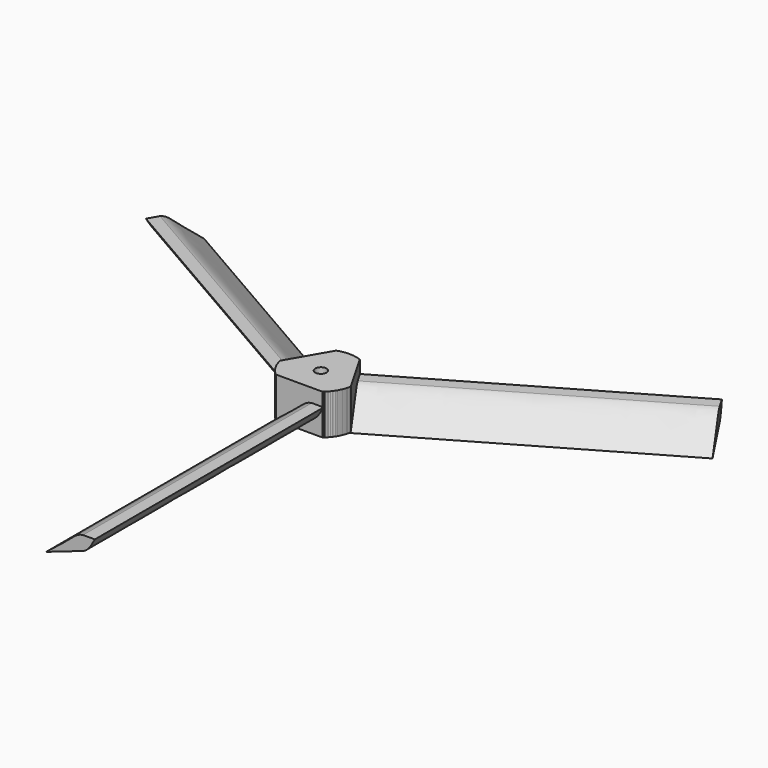
from build123d import *

# Parameters (mm, degrees)
F0_R     = 6.35
F0_R_2   = 0.99949
F1_DEPTH = 9.525
F4_DEPTH = 25.4
F6_DEPTH = 50.8
F7_COUNT = 3
F8_W     = 8.2890069642
F8_H     = 2.380754333
F9_DEPTH = 25.4


with BuildPart() as f1:
    # F0 (on Top) → F1 (new body)
    with BuildSketch(Plane.XY):
        Circle(F0_R)
        Circle(F0_R_2, mode=Mode.SUBTRACT)
    extrude(amount=F1_DEPTH)

    # F3 (on offset) → F4 (cut)
    with BuildSketch(Plane.XY.offset(9.525)):
        Polygon((-19.2380820383, -11.0045537162), (19.2410791448, -11.0045537162), (0.0014985533, 22.3193773847), align=None)
        Polygon((0.0014985533, 9.6193773847), (8.2425565167, -4.6545537162), (-8.2395594102, -4.6545537162), (-8.2425565167, -4.6545537162), (0, 9.621972955), align=None, mode=Mode.SUBTRACT)
    extrude(amount=-F4_DEPTH, mode=Mode.SUBTRACT)

    # F5 (on face) → F6 (join)
    with BuildSketch(Plane.XZ.offset(4.6545537162)):
        with BuildLine():
            add(Edge.make_bspline(
                [(4.319447847, 7.14375), (3.8768217141, 6.3398531681), (3.0702504394, 4.8749597867), (1.3331871276, 4.307573582), (-1.2552066512, 3.4811706955), (-3.2623562204, 2.7606969439), (-4.319447847, 2.38125)],
                knots=[0, 0, 0, 0, 0.2497283334, 0.4550650881, 0.7130028867, 1, 1, 1, 1], degree=3))
            Line((4.319447847, 7.14375), (2.2289671052, 7.14375))
            add(Edge.make_bspline(
                [(2.2289671052, 7.14375), (2.0794537401, 7.1223183312), (1.3375273881, 6.9699970017), (0.3270313355, 6.1326811809), (-1.7535535369, 4.3851427196), (-3.4342742537, 3.0725461739), (-4.319447847, 2.38125)],
                knots=[0.2009623726, 0.2009623726, 0.2009623726, 0.2009623726, 0.2497283334, 0.4550650881, 0.7130028867, 1, 1, 1, 1], degree=3))
        make_face()
    extrude(amount=F6_DEPTH)


with BuildPart() as f7_1:
    # F7: instance of F1
    add(f1.part.rotate(Axis((0, 0, 9.525), (0, 0, 1)), 1 * 360 / F7_COUNT))


with BuildPart() as f7_2:
    # F7: instance of F1
    add(f1.part.rotate(Axis((0, 0, 9.525), (0, 0, 1)), 2 * 360 / F7_COUNT))


with BuildPart() as f9_tool:
    # F8 (on face) → F9 (new body)
    with BuildSketch(Plane.XZ.offset(4.8109864775)):
        Polygon((-4.1445034821, 2.380754333), (-6.2417029403, 2.380754333), (-6.2417029403, -0.2239797032), (6.5267146565, -0.2239797032), (6.5267146565, 2.380754333), (4.1445034821, 2.380754333), (4.1445034821, 0), (-4.1445034821, 0), align=None)
        with Locations((0, 1.1903771665)):
            Rectangle(F8_W, F8_H)
    extrude(amount=-F9_DEPTH)


with BuildPart() as f1_1:
    add(f1.part)

    # F9: cut by f9_tool
    add(f9_tool.part, mode=Mode.SUBTRACT)


with BuildPart() as f7_1_1:
    add(f7_1.part)

    # F9: cut by f9_tool
    add(f9_tool.part, mode=Mode.SUBTRACT)


with BuildPart() as f7_2_1:
    add(f7_2.part)

    # F9: cut by f9_tool
    add(f9_tool.part, mode=Mode.SUBTRACT)


solid = Compound([f1_1.part, f7_1_1.part, f7_2_1.part])
